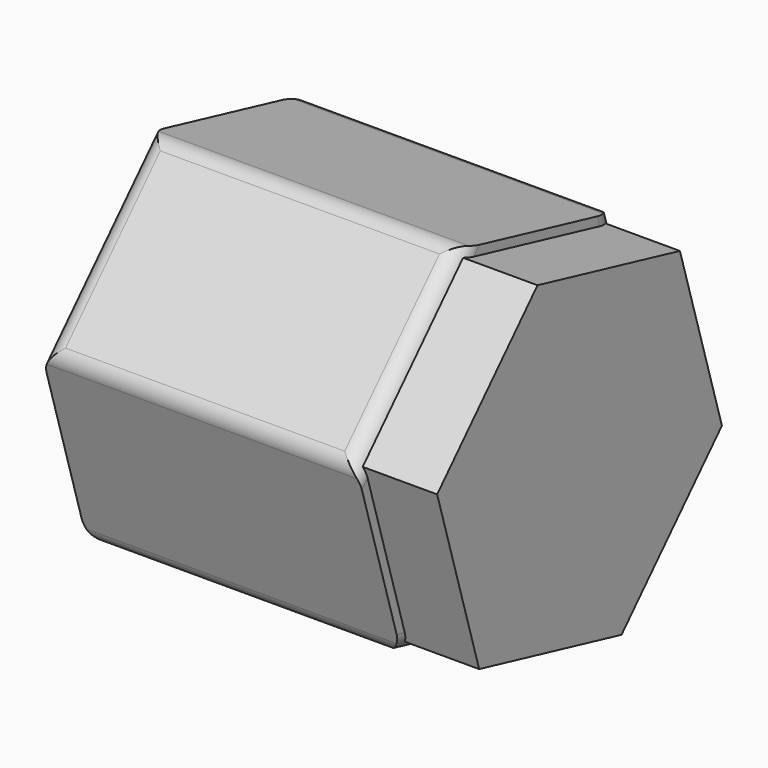
from build123d import *

# Parameters (mm, degrees)
F1_DEPTH    = 88.9
F2_T        = -2.54
F3_T1_DEPTH = 103.5646968374
F3_T3_DEPTH = 79.9330955154
F4_T1_DEPTH = 103.5646968374
F4_T3_DEPTH = 79.9330955154
F5_T1_DEPTH = 103.5646968374
F5_T3_DEPTH = 79.9330955154
F6_DEPTH    = 22.86


# Not quite as in the source:
# - a fillet or chamfer that OpenCascade refuses, or shapes differently, is made with other operations: its cross-section is extruded or revolved along the edge and cut away or added


with BuildPart() as f1:
    # F0 (on Right) → F1 (new body)
    with BuildSketch(Plane.YZ):
        Polygon((-15.657663601, 52.2369225457), (-53.0673337406, 12.5585268304), (-37.4096701396, -39.6783957152), (15.657663601, -52.2369225457), (53.0673337406, -12.5585268304), (37.4096701396, 39.6783957152), align=None)
    extrude(amount=F1_DEPTH)

    # F2
    f2_openings = [f1.faces().sort_by_distance(p)[0] for p in [
        (0, 0, 0),
    ]]
    offset(amount=F2_T, openings=f2_openings)

    # F3: fillet of radius 5.08 on 4 edges, made by hand

    # F3_s2 → F3_t1 (cut)
    with BuildSketch(Plane.YZ.offset(-7.3323484187)):
        with BuildLine():
            ThreePointArc((-12.8035569199, 51.5614905463), (-15.4320203518, 51.484134056), (-17.6696582116, 50.1029096544))
            Line((-17.6696582116, 50.1029096544), (-15.657663601, 52.2369225457))
            Line((-15.657663601, 52.2369225457), (-12.8035569199, 51.5614905463))
        make_face()
        with BuildLine():
            ThreePointArc((-51.05533913, 14.6925397217), (-52.3025781603, 12.3775453716), (-52.22522167, 9.7490819397))
            Line((-52.22522167, 9.7490819397), (-53.0673337406, 12.5585268304))
            Line((-53.0673337406, 12.5585268304), (-51.05533913, 14.6925397217))
        make_face()
    extrude(amount=F3_T1_DEPTH, mode=Mode.SUBTRACT)

    # F3_s4 → F3_t3 (cut)
    with BuildSketch(Plane(origin=(0, 27.4170272951, 29.0797447369), x_dir=(1, 0, 0), z_dir=(0, -0.6859993878, -0.7276021165))):
        with BuildLine():
            ThreePointArc((5.08, 47.2270460633), (1.4878975516, 45.7391485117), (0, 42.1470460633))
            Line((0, 42.1470460633), (0, 47.2270460633))
            Line((0, 47.2270460633), (5.08, 47.2270460633))
        make_face()
        with BuildLine():
            ThreePointArc((83.82, 47.2270460633), (87.4121024484, 45.7391485117), (88.9, 42.1470460633))
            Line((88.9, 42.1470460633), (88.9, 47.2270460633))
            Line((88.9, 47.2270460633), (83.82, 47.2270460633))
        make_face()
    extrude(amount=F3_T3_DEPTH, mode=Mode.SUBTRACT)

    # F4: fillet of radius 5.08 on 4 edges, made by hand

    # F4_s2 → F4_t1 (cut)
    with BuildSketch(Plane.YZ.offset(-7.3323484187)):
        with BuildLine():
            ThreePointArc((52.22522167, -9.7490819397), (52.3025781603, -12.3775453716), (51.05533913, -14.6925397217))
            Line((51.05533913, -14.6925397217), (53.0673337406, -12.5585268304))
            Line((53.0673337406, -12.5585268304), (52.22522167, -9.7490819397))
        make_face()
        with BuildLine():
            ThreePointArc((38.2517822101, 36.8689508245), (36.8705578085, 39.1065886844), (34.5555634584, 40.3538277147))
            Line((34.5555634584, 40.3538277147), (37.4096701396, 39.6783957152))
            Line((37.4096701396, 39.6783957152), (38.2517822101, 36.8689508245))
        make_face()
    extrude(amount=F4_T1_DEPTH, mode=Mode.SUBTRACT)

    # F4_s4 → F4_t3 (cut)
    with BuildSketch(Plane(origin=(0, 11.4752840302, -38.2837145023), x_dir=(1, 0, 0), z_dir=(0, -0.2871222228, 0.9578939551))):
        with BuildLine():
            ThreePointArc((5.08, 47.2270460633), (1.4878975516, 45.7391485117), (0, 42.1470460633))
            Line((0, 42.1470460633), (0, 47.2270460633))
            Line((0, 47.2270460633), (5.08, 47.2270460633))
        make_face()
        with BuildLine():
            ThreePointArc((83.82, 47.2270460633), (87.4121024484, 45.7391485117), (88.9, 42.1470460633))
            Line((88.9, 42.1470460633), (88.9, 47.2270460633))
            Line((88.9, 47.2270460633), (83.82, 47.2270460633))
        make_face()
    extrude(amount=F4_T3_DEPTH, mode=Mode.SUBTRACT)

    # F5: fillet of radius 5.08 on 4 edges, made by hand

    # F5_s2 → F5_t1 (cut)
    with BuildSketch(Plane.YZ.offset(-7.3323484187)):
        with BuildLine():
            ThreePointArc((-34.5555634584, -40.3538277147), (-36.8705578085, -39.1065886844), (-38.2517822101, -36.8689508245))
            Line((-38.2517822101, -36.8689508245), (-37.4096701396, -39.6783957152))
            Line((-37.4096701396, -39.6783957152), (-34.5555634584, -40.3538277147))
        make_face()
        with BuildLine():
            ThreePointArc((17.6696582116, -50.1029096544), (15.4320203518, -51.484134056), (12.8035569199, -51.5614905463))
            Line((12.8035569199, -51.5614905463), (15.657663601, -52.2369225457))
            Line((15.657663601, -52.2369225457), (17.6696582116, -50.1029096544))
        make_face()
    extrude(amount=F5_T1_DEPTH, mode=Mode.SUBTRACT)

    # F5_s4 → F5_t3 (cut)
    with BuildSketch(Plane(origin=(0, -38.8923113253, 9.2039697654), x_dir=(1, 0, 0), z_dir=(0, 0.9731216106, -0.2302918386))):
        with BuildLine():
            ThreePointArc((0, 42.1470460633), (1.4878975516, 45.7391485117), (5.08, 47.2270460633))
            Line((5.08, 47.2270460633), (0, 47.2270460633))
            Line((0, 47.2270460633), (0, 42.1470460633))
        make_face()
        with BuildLine():
            ThreePointArc((88.9, 42.1470460633), (87.4121024484, 45.7391485117), (83.82, 47.2270460633))
            Line((83.82, 47.2270460633), (88.9, 47.2270460633))
            Line((88.9, 47.2270460633), (88.9, 42.1470460633))
        make_face()
    extrude(amount=F5_T3_DEPTH, mode=Mode.SUBTRACT)

    # F6 (add): a face of the model
    f6_faces = [f1.faces().sort_by_distance(p)[0] for p in [
        (86.36, 0, 0),
    ]]
    extrude(f6_faces, amount=-F6_DEPTH)


solid = f1.part
